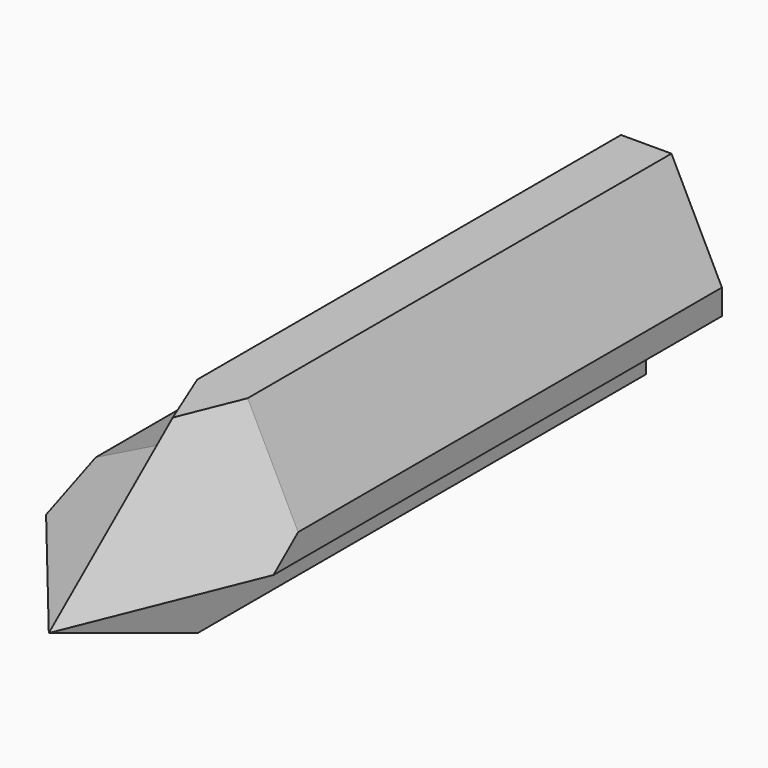
from build123d import *

# Parameters (mm, degrees)
F1_DEPTH    = 762
F2_T1_DEPTH = 1300.1781500313
F2_T3_DEPTH = 1300.1781500313
F4_ANGLE    = 90


# Not quite as in the source:
# - a fillet or chamfer that OpenCascade refuses, or shapes differently, is made with other operations: its cross-section is extruded or revolved along the edge and cut away or added


with BuildPart() as f1:
    # F0 (on Front) → F1 (new body)
    with BuildSketch(Plane.XZ):
        Polygon((0, -76.2), (0, 76.2), (-25.4, 76.2), (-127.5811195374, 25.4), (-127.5811195374, 0), (-127.5811195374, -25.4), (-25.4, -76.2), align=None)
    extrude(amount=F1_DEPTH)

    # F2: chamfer of 228.6 x 83.2035955533 on 2 edges, made by hand

    # F2_s2 → F2_t1 (cut)
    with BuildSketch(Plane(origin=(541.036756959, 0, 268.9798993978), x_dir=(0, 1, 0), z_dir=(-0.8954433759, 0, -0.4451754267))):
        Polygon((-762, 3.6633544712), (-533.4, -79.540241082), (-762, -79.540241082), align=None)
    extrude(amount=F2_T1_DEPTH, mode=Mode.SUBTRACT)

    # F2_s4 → F2_t3 (cut)
    with BuildSketch(Plane(origin=(-623.1991549624, 0, 309.8274633849), x_dir=(0, 1, 0), z_dir=(0.8954433759, 0, -0.4451754267))):
        Polygon((-533.4, -79.540241082), (-762, 3.6633544712), (-762, -79.540241082), align=None)
    extrude(amount=F2_T3_DEPTH, mode=Mode.SUBTRACT)


with BuildPart() as f4_1:
    # F4: copy of F1
    add(f1.part.rotate(Axis((0, -626.9350163109, 0), (0, 1, 0)), F4_ANGLE))


solid = Compound([f1.part, f4_1.part])
